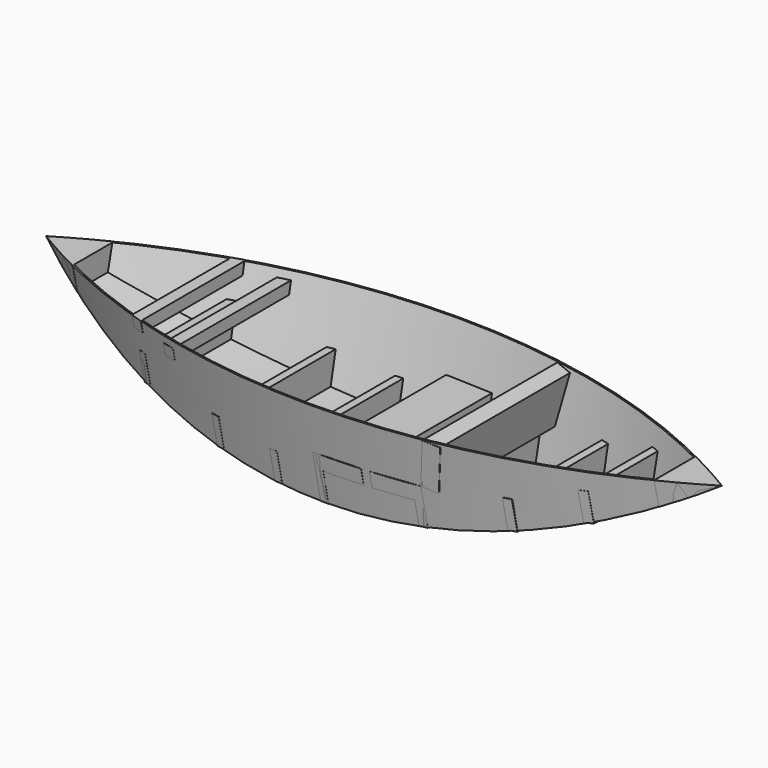
from build123d import *

# Parameters (mm, degrees)
F1_DEPTH               = 609.6
F2_W                   = 2380.1591098309
F2_H                   = 883.9359134436
F3_DEPTH               = 508
DRAFT_F3_DRAFTED_ANGLE = -12
F4_T                   = 5.159375
F6_DEPTH               = 762
F5_W                   = 38.1
F5_H                   = 38.1
F7_W                   = 2307.9005777836
F7_H                   = 882.3253214359
F8_DEPTH               = 508
DRAFT_F8_DRAFTED_ANGLE = -12


# Not quite as in the source:
# - an extrude with a draft is written as a straight extrude whose walls are then drafted
# - a shell that OpenCascade refuses in one call is made with other operations: the cavity is built on its own and cut out


with BuildPart() as f1:
    # F0 (on Front) → F1 (new body)
    with BuildSketch(Plane.XZ):
        with BuildLine():
            Line((2184.4, 0), (0, 0))
            ThreePointArc((0, 0), (1092.2, -304.8), (2184.4, 0))
        make_face()
    extrude(amount=-F1_DEPTH)


with BuildPart() as f3_drafted:
    # F2 (on face) → F3 (new body)
    with BuildSketch(Plane.XY):
        with Locations((1096.2463766336, 278.8261845708)):
            Rectangle(F2_W, F2_H)
        with BuildLine():
            ThreePointArc((2184.4, 304.8), (1092.2, 0), (0, 304.8))
            ThreePointArc((0, 304.8), (1092.2, 609.6), (2184.4, 304.8))
        make_face(mode=Mode.SUBTRACT)
    extrude(amount=-F3_DEPTH)

    # draft_F3_drafted
    draft_f3_drafted_walls = [f3_drafted.faces().sort_by_distance(p)[0] for p in [
        (1096.2463766336, 720.7941412926, -338.6666666667),
        (-93.8331782818, 278.8261845708, -338.6666666667),
        (1096.2463766336, -163.141772151, -338.6666666667),
        (2286.3259315491, 278.8261845708, -338.6666666667),
        (1092.2, 0, -338.6666666667),
        (1092.2, 609.6, -338.6666666667),
    ]]
    draft(draft_f3_drafted_walls, neutral_plane=Plane(origin=(0, 0, 0), x_dir=(1, 0, 0), z_dir=(0, 0, -1)), angle=DRAFT_F3_DRAFTED_ANGLE)


with BuildPart() as f1_1:
    add(f1.part)

    # join_F3_drafted: cut F3_drafted
    add(f3_drafted.part, mode=Mode.SUBTRACT)

    # F4: shell of thickness 5.159375, made by hand


with BuildPart() as f4_core1:
    # F4_t2: copy of F1
    add(f1_1.part)

    # the walls: a layer under each face that stays
    f4_faces = [f4_core1.faces().sort_by_distance(p)[0] for p in [
        (1092.2, 577.2017535498, -152.4217657441),
        (1092.2, 304.8, -304.8),
        (1092.2, 32.3982464502, -152.4217657441),
    ]]
    thicken(f4_faces, amount=-F4_T, mode=Mode.SUBTRACT)


with BuildPart() as f1_2:
    add(f1_1.part)

    # what is left inside the walls is the cavity
    f4_cavity = [f4_core1.part.solids().sort_by_distance(p)[0] for p in [
        (1092.2, 404.641787, -0.051594),
    ]]
    add(f4_cavity, mode=Mode.SUBTRACT)


with BuildPart() as f6:
    # F5 (on Front) → F6 (new body)
    with BuildSketch(Plane.XZ):
        with BuildLine():
            Line((1079.501807367, -304.7617767168), (1079.501807367, -304.7999999992))
            Line((1079.501807367, -304.7999999992), (1092.2, -304.7999999992))
            ThreePointArc((1092.2, -304.8), (1085.8508749192, -304.7904441576), (1079.5018073669, -304.7617767168))
        make_face()
        with BuildLine():
            ThreePointArc((1104.901807367, -304.7617549518), (1098.5509324723, -304.7904387163), (1092.2, -304.8))
            Line((1092.2, -304.7999999992), (1104.901807367, -304.7999999992))
            Line((1104.901807367, -304.7999999992), (1104.901807367, -304.7617549518))
        make_face()
        with BuildLine():
            ThreePointArc((1079.5018073669, -304.7617767168), (1085.8508749192, -304.7904441576), (1092.2, -304.8))
            ThreePointArc((1092.2, -304.8), (1098.5509324723, -304.7904387163), (1104.901807367, -304.7617549518))
            Line((1104.901807367, -304.7617549518), (1104.901807367, -203.1999999992))
            Line((1104.901807367, -203.1999999992), (1079.501807367, -203.1999999992))
            Line((1079.501807367, -203.1999999992), (1079.501807367, -304.7617767168))
        make_face()
        Polygon((1079.501807367, -152.3999999992), (1079.501807367, -203.1999999992), (1104.901807367, -203.1999999992), (1231.901807367, -203.1999999992), (1231.901807367, -152.3999999992), align=None)
    extrude(amount=-F6_DEPTH)


with BuildPart() as f6b:
    # F5 (on Front) → F6, piece 2 (new body)
    with BuildSketch(Plane.XZ):
        with BuildLine():
            ThreePointArc((0, 0), (75.3351461515, -43.5017814267), (152.4, -83.8601452968))
            Line((152.4, -83.8601452968), (152.4, 0))
            Line((152.4, 0), (0, 0))
        make_face()
    extrude(amount=-F6_DEPTH)


with BuildPart() as f6c:
    # F5 (on Front) → F6, piece 3 (new body)
    with BuildSketch(Plane.XZ):
        with BuildLine():
            Line((444.5082454406, -206.9481865869), (457.2082454407, -206.9481865869))
            ThreePointArc((457.2082454407, -206.948186587), (450.8550429945, -204.931465302), (444.5082454407, -202.8946769297))
            Line((444.5082454406, -202.8946769297), (444.5082454406, -206.9481865869))
        make_face()
        with BuildLine():
            ThreePointArc((444.5082454407, -202.8946769297), (450.8550429945, -204.931465302), (457.2082454407, -206.948186587))
            Line((457.2082454407, -206.9481865869), (469.9082454406, -206.9481865869))
            Line((469.9082454406, -206.9481865869), (469.9082454406, -105.3481865869))
            Line((469.9082454406, -105.3481865869), (444.5082454406, -105.3481865869))
            Line((444.5082454406, -105.3481865869), (444.5082454406, -202.8946769297))
        make_face()
    extrude(amount=-F6_DEPTH)


with BuildPart() as f6d:
    # F5 (on Front) → F6, piece 4 (new body)
    with BuildSketch(Plane.XZ):
        with BuildLine():
            Line((723.901807367, -274.608919579), (736.601807367, -274.608919579))
            ThreePointArc((736.601807367, -274.608919579), (730.250117362, -273.5125517357), (723.901807367, -272.3967790997))
            Line((723.901807367, -272.3967790997), (723.901807367, -274.608919579))
        make_face()
        with BuildLine():
            ThreePointArc((723.901807367, -272.3967790997), (730.250117362, -273.5125517357), (736.601807367, -274.608919579))
            Line((736.601807367, -274.608919579), (749.301807367, -274.608919579))
            Line((749.301807367, -274.608919579), (749.301807367, -173.008919579))
            Line((749.301807367, -173.008919579), (723.901807367, -173.008919579))
            Line((723.901807367, -173.008919579), (723.901807367, -272.3967790997))
        make_face()
    extrude(amount=-F6_DEPTH)


with BuildPart() as f6e:
    # F5 (on Front) → F6, piece 5 (new body)
    with BuildSketch(Plane.XZ):
        with BuildLine():
            Line((927.101807367, -299.287256708), (939.8018073668, -299.287256708))
            ThreePointArc((939.8018073668, -299.287256708), (933.4510838699, -298.8175635389), (927.101807367, -298.3286990419))
            Line((927.101807367, -298.3286990419), (927.101807367, -299.287256708))
        make_face()
        with BuildLine():
            ThreePointArc((927.101807367, -298.3286990419), (933.4510838699, -298.8175635389), (939.8018073668, -299.287256708))
            Line((939.8018073668, -299.287256708), (952.501807367, -299.287256708))
            Line((952.501807367, -299.287256708), (952.501807367, -197.687256708))
            Line((952.501807367, -197.687256708), (927.101807367, -197.687256708))
            Line((927.101807367, -197.687256708), (927.101807367, -298.3286990419))
        make_face()
    extrude(amount=-F6_DEPTH)


with BuildPart() as f6f:
    # F5 (on Front) → F6, piece 6 (new body)
    with BuildSketch(Plane.XZ):
        Polygon((1436.1639822764, -2.3152984402), (1409.7, -152.3999999992), (1459.728233853, -161.2213274247), (1486.1922161295, -11.1366258656), align=None)
    extrude(amount=-F6_DEPTH)


with BuildPart() as f6g:
    # F5 (on Front) → F6, piece 7 (new body)
    with BuildSketch(Plane.XZ):
        with BuildLine():
            Line((2032, 0), (2032, -83.8601452968))
            ThreePointArc((2032, -83.8601452968), (2109.0648538485, -43.5017814267), (2184.4, 0))
            Line((2184.4, 0), (2032, 0))
        make_face()
    extrude(amount=-F6_DEPTH)


with BuildPart() as f6h:
    # F5 (on Front) → F6, piece 8 (new body)
    with BuildSketch(Plane.XZ):
        with BuildLine():
            Line((1841.5, -162.347889134), (1854.2000000001, -162.347889134))
            ThreePointArc((1854.2000000001, -162.3478891339), (1860.5540146702, -159.8743332169), (1866.9, -157.3802499186))
            Line((1866.9, -157.3802499186), (1866.9, -60.747889134))
            Line((1866.9, -60.747889134), (1841.5, -60.747889134))
            Line((1841.5, -60.747889134), (1841.5, -162.347889134))
        make_face()
        with BuildLine():
            ThreePointArc((1866.9, -157.3802499186), (1860.5540146702, -159.8743332169), (1854.2000000001, -162.3478891339))
            Line((1854.2000000001, -162.347889134), (1866.9, -162.347889134))
            Line((1866.9, -162.347889134), (1866.9, -157.3802499186))
        make_face()
    extrude(amount=-F6_DEPTH)


with BuildPart() as f6i:
    # F5 (on Front) → F6, piece 9 (new body)
    with BuildSketch(Plane.XZ):
        with BuildLine():
            Line((1638.3, -229.4328330608), (1651.0000000001, -229.4328330608))
            ThreePointArc((1651.0000000001, -229.4328330608), (1657.3527591748, -227.6767693439), (1663.7, -225.9008631479))
            Line((1663.7, -225.9008631479), (1663.7, -127.8328330608))
            Line((1663.7, -127.8328330608), (1638.3, -127.8328330608))
            Line((1638.3, -127.8328330608), (1638.3, -229.4328330608))
        make_face()
        with BuildLine():
            ThreePointArc((1663.7, -225.9008631479), (1657.3527591748, -227.6767693439), (1651.0000000001, -229.4328330608))
            Line((1651.0000000001, -229.4328330608), (1663.7, -229.4328330608))
            Line((1663.7, -229.4328330608), (1663.7, -225.9008631479))
        make_face()
    extrude(amount=-F6_DEPTH)


with BuildPart() as f6j:
    # F5 (on Front) → F6, piece 10 (new body)
    with BuildSketch(Plane.XZ):
        with BuildLine():
            Line((1384.3, -282.6611353929), (1397, -282.6611353929))
            ThreePointArc((1397, -282.6611353929), (1403.3514414045, -281.723705044), (1409.7, -280.7669462794))
            Line((1409.7, -280.7669462794), (1409.7, -203.1999999992))
            Line((1409.7, -203.1999999992), (1384.3, -203.1999999992))
            Line((1384.3, -203.1999999992), (1384.3, -282.6611353929))
        make_face()
        with BuildLine():
            ThreePointArc((1409.7, -280.7669462794), (1403.3514414045, -281.723705044), (1397, -282.6611353929))
            Line((1397, -282.6611353929), (1409.7, -282.6611353929))
            Line((1409.7, -282.6611353929), (1409.7, -280.7669462794))
        make_face()
        Polygon((1384.3, -203.1999999992), (1409.7, -203.1999999992), (1409.7, -152.3999999992), (1257.3, -152.3999999992), (1257.3, -203.1999999992), align=None)
    extrude(amount=-F6_DEPTH)


with BuildPart() as f6k:
    # F5 (on Front) → F6, piece 11 (new body)
    with BuildSketch(Plane.XZ):
        with Locations((457.2082454406, -19.05)):
            Rectangle(F5_W, F5_H)
    extrude(amount=-F6_DEPTH)


with BuildPart() as f6l:
    # F5 (on Front) → F6, piece 12 (new body)
    with BuildSketch(Plane.XZ):
        with Locations((584.201807367, -44.45)):
            Rectangle(F5_W, F5_H)
    extrude(amount=-F6_DEPTH)


with BuildPart() as f8_drafted:
    # F7 (on Top) → F8 (new body)
    with BuildSketch(Plane.XY):
        with Locations((1103.4626215696, 367.1494573355)):
            Rectangle(F7_W, F7_H)
        with BuildLine():
            ThreePointArc((0, 304.8), (1092.2, 609.6), (2184.4, 304.8))
            ThreePointArc((2184.4, 304.8), (1092.2, 0), (0, 304.8))
        make_face(mode=Mode.SUBTRACT)
    extrude(amount=-F8_DEPTH)

    # draft_F8_drafted
    draft_f8_drafted_walls = [f8_drafted.faces().sort_by_distance(p)[0] for p in [
        (1103.4626215696, 808.3121180534, -338.6666666667),
        (-50.4876673222, 367.1494573355, -338.6666666667),
        (1103.4626215696, -74.0132033825, -338.6666666667),
        (2257.4129104614, 367.1494573355, -338.6666666667),
        (1092.2, 0, -338.6666666667),
        (1092.2, 609.6, -338.6666666667),
    ]]
    draft(draft_f8_drafted_walls, neutral_plane=Plane(origin=(0, 0, 0), x_dir=(1, 0, 0), z_dir=(0, 0, -1)), angle=DRAFT_F8_DRAFTED_ANGLE)


with BuildPart() as f6_1:
    add(f6.part)

    # join_F8_drafted: cut F8_drafted
    add(f8_drafted.part, mode=Mode.SUBTRACT)


with BuildPart() as f6b_1:
    add(f6b.part)

    # join_F8_drafted: cut F8_drafted
    add(f8_drafted.part, mode=Mode.SUBTRACT)


with BuildPart() as f6c_1:
    add(f6c.part)

    # join_F8_drafted: cut F8_drafted
    add(f8_drafted.part, mode=Mode.SUBTRACT)


with BuildPart() as f6d_1:
    add(f6d.part)

    # join_F8_drafted: cut F8_drafted
    add(f8_drafted.part, mode=Mode.SUBTRACT)


with BuildPart() as f6e_1:
    add(f6e.part)

    # join_F8_drafted: cut F8_drafted
    add(f8_drafted.part, mode=Mode.SUBTRACT)


with BuildPart() as f6f_1:
    add(f6f.part)

    # join_F8_drafted: cut F8_drafted
    add(f8_drafted.part, mode=Mode.SUBTRACT)


with BuildPart() as f6g_1:
    add(f6g.part)

    # join_F8_drafted: cut F8_drafted
    add(f8_drafted.part, mode=Mode.SUBTRACT)


with BuildPart() as f6h_1:
    add(f6h.part)

    # join_F8_drafted: cut F8_drafted
    add(f8_drafted.part, mode=Mode.SUBTRACT)


with BuildPart() as f6i_1:
    add(f6i.part)

    # join_F8_drafted: cut F8_drafted
    add(f8_drafted.part, mode=Mode.SUBTRACT)


with BuildPart() as f6j_1:
    add(f6j.part)

    # join_F8_drafted: cut F8_drafted
    add(f8_drafted.part, mode=Mode.SUBTRACT)


with BuildPart() as f6k_1:
    add(f6k.part)

    # join_F8_drafted: cut F8_drafted
    add(f8_drafted.part, mode=Mode.SUBTRACT)


with BuildPart() as f6l_1:
    add(f6l.part)

    # join_F8_drafted: cut F8_drafted
    add(f8_drafted.part, mode=Mode.SUBTRACT)


solid = Compound([f1_2.part, f6_1.part, f6b_1.part, f6c_1.part, f6d_1.part, f6e_1.part, f6f_1.part, f6g_1.part, f6h_1.part, f6i_1.part, f6j_1.part, f6k_1.part, f6l_1.part])
